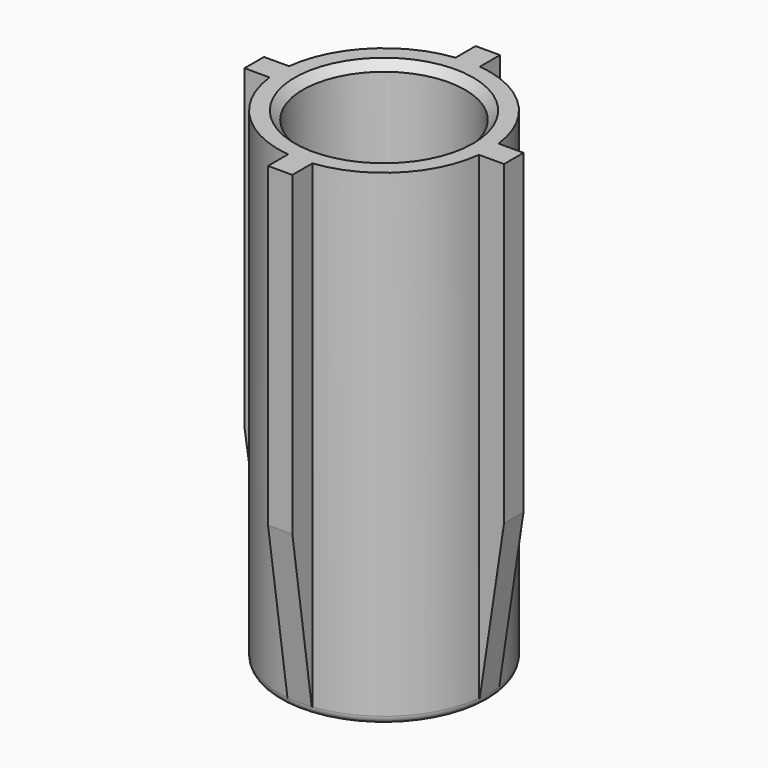
from build123d import *

# Parameters (mm, degrees)
F1_R        = 6.5
F1_R_2      = 5
F2_DEPTH    = 30
F4_W        = 1.5
F4_H        = 2.639524132
F5_DEPTH    = 29.5
F6_COUNT    = 4
F8_R        = 5
F8_R_2      = 2.75
F9_DEPTH    = 1.5
F10_SIZE2   = 1.49999
F10_SIZE    = 9.99999
F10_2_SIZE2 = 1.49999
F10_2_SIZE  = 9.99999
F10_3_SIZE2 = 1.49999
F10_3_SIZE  = 9.99999
F10_4_SIZE2 = 1.49999
F10_4_SIZE  = 9.99999
F11_SIZE    = 0.5
F12_R       = 0.49999


# Not quite as in the source:
# - a fillet or chamfer is up to 0.001 mm smaller than in the source, because OpenCascade refuses the exact size


with BuildPart() as f2:
    # F1 (on offset) → F2 (new body)
    with BuildSketch(Plane.XY):
        with Locations((-25, 25)):
            Circle(F1_R)
        with Locations((-25, 25)):
            Circle(F1_R_2, mode=Mode.SUBTRACT)
    extrude(amount=-F2_DEPTH)

    # F4 (on offset) → F5 (join)
    with BuildSketch(Plane.XY):
        with Locations((-25, 31.680237934)):
            Rectangle(F4_W, F4_H)
    extrude(amount=-F5_DEPTH)

    # F6: F2 ×4 about axis
    f6_axis = Axis((-25, 25, 0), (0, 0, 1))


with BuildPart() as f2_1:
    add(f2.part)
    for i in range(1, F6_COUNT):
        add(f2.part.rotate(f6_axis, i * 360 / F6_COUNT))

    # F8 (on offset) → F9 (join)
    with BuildSketch(Plane.XY.offset(-30)):
        with Locations((-25, 25)):
            Circle(F8_R)
        with Locations((-25, 25)):
            Circle(F8_R_2, mode=Mode.SUBTRACT)
    extrude(amount=F9_DEPTH)

    # F10 (size 10 and 1.5 in the source; OpenCascade refuses exactly that, so slightly less here)
    f10_edges = [f2_1.edges().sort_by_distance(p)[0] for p in [
        (-25, 17, -29.5),
    ]]
    f10_side = f2_1.faces().sort_by_distance((-25, 17, -14.75))[0]
    chamfer(f10_edges, length=F10_SIZE, length2=F10_SIZE2, reference=f10_side)

    # F10#2 (size 10 and 1.5 in the source; OpenCascade refuses exactly that, so slightly less here)
    f10_2_edges = [f2_1.edges().sort_by_distance(p)[0] for p in [
        (-17, 25, -29.5),
    ]]
    f10_2_side = f2_1.faces().sort_by_distance((-17, 25, -14.75))[0]
    chamfer(f10_2_edges, length=F10_2_SIZE, length2=F10_2_SIZE2, reference=f10_2_side)

    # F10#3 (size 10 and 1.5 in the source; OpenCascade refuses exactly that, so slightly less here)
    f10_3_edges = [f2_1.edges().sort_by_distance(p)[0] for p in [
        (-25, 33, -29.5),
    ]]
    f10_3_side = f2_1.faces().sort_by_distance((-25, 33, -14.75))[0]
    chamfer(f10_3_edges, length=F10_3_SIZE, length2=F10_3_SIZE2, reference=f10_3_side)

    # F10#4 (size 10 and 1.5 in the source; OpenCascade refuses exactly that, so slightly less here)
    f10_4_edges = [f2_1.edges().sort_by_distance(p)[0] for p in [
        (-33, 25, -29.5),
    ]]
    f10_4_side = f2_1.faces().sort_by_distance((-33, 25, -14.75))[0]
    chamfer(f10_4_edges, length=F10_4_SIZE, length2=F10_4_SIZE2, reference=f10_4_side)

    # F11
    f11_edges = [f2_1.edges().sort_by_distance(p)[0] for p in [
        (-30, 25, 0),
        (-27.75, 25, -28.5),
    ]]
    chamfer(f11_edges, length=F11_SIZE)

    # F12 (radius 0.5 in the source; OpenCascade refuses exactly that, so slightly less here)
    f12_edges = [f2_1.edges().sort_by_distance(p)[0] for p in [
        (-31.5, 25, -30),
    ]]
    fillet(f12_edges, radius=F12_R)


solid = f2_1.part
